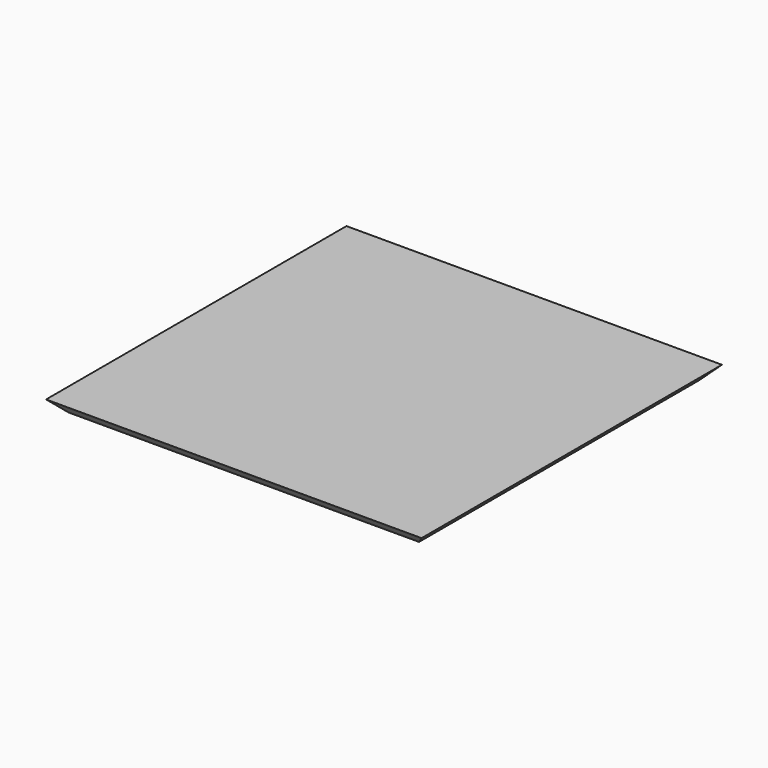
from build123d import *

# Parameters (mm, degrees)
F0_W     = 76.2
F0_H     = 76.2
F1_DEPTH = 2.54
F2_SIZE  = 2.53999


# Not quite as in the source:
# - a fillet or chamfer is up to 0.001 mm smaller than in the source, because OpenCascade refuses the exact size


with BuildPart() as f1:
    # F0 (on Top) → F1 (new body)
    with BuildSketch(Plane.XY):
        with Locations((38.1, 38.1)):
            Rectangle(F0_W, F0_H)
    extrude(amount=F1_DEPTH)

    # F2 (size 2.54 in the source; OpenCascade refuses exactly that, so slightly less here)
    f2_edges = [f1.edges().sort_by_distance(p)[0] for p in [
        (0, 38.1, 0),
        (38.1, 0, 0),
        (76.2, 38.1, 0),
        (38.1, 76.2, 0),
    ]]
    chamfer(f2_edges, length=F2_SIZE)


solid = f1.part
